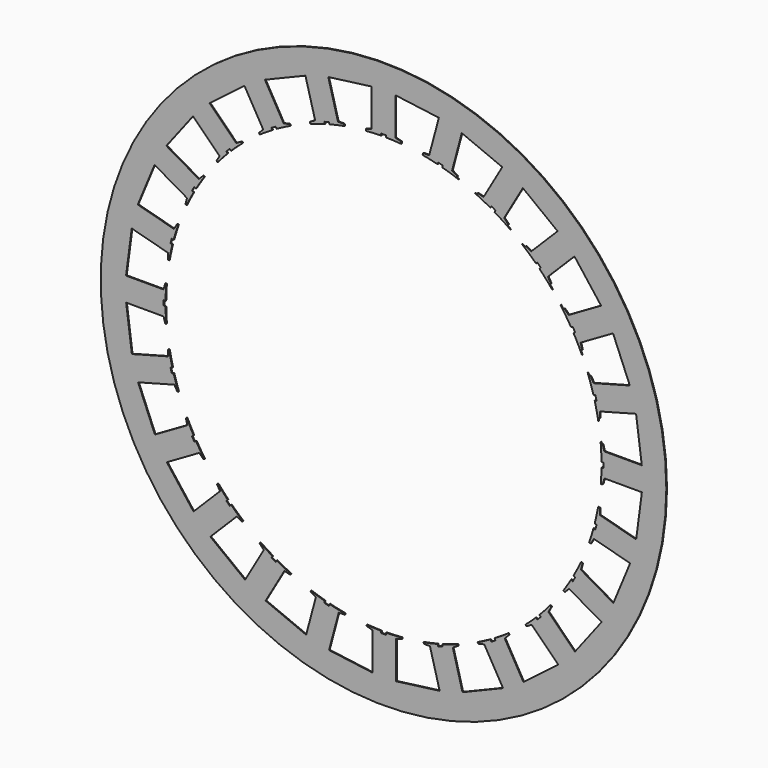
from build123d import *

# Parameters (mm, degrees)
F0_R     = 117.42
F0_R_2   = 90.5
F1_DEPTH = 0.35
F3_DEPTH = 0.351
F5_DEPTH = 0.351


with BuildPart() as f1:
    # F0 (on Front) → F1 (new body)
    with BuildSketch(Plane.XZ):
        Circle(F0_R)
        Circle(F0_R_2, mode=Mode.SUBTRACT)
    extrude(amount=F1_DEPTH)

    # F2 (on face) → F3 (cut, through all)
    with BuildSketch(Plane.XZ.offset(0.35)):
        with BuildLine():
            Line((7.35, 91.001039351), (7.35, 90.201039351))
            ThreePointArc((7.35, 90.201039351), (11.8126203959, 89.7257599543), (16.2461920489, 89.0298334487))
            Line((16.2461920489, 89.0298334487), (16.4532472849, 89.8025741098))
            Line((16.4532472849, 89.8025741098), (18.9519490961, 89.8163312564))
            Line((18.9519490961, 89.8163312564), (22.9791734379, 104.8461371135))
            Line((22.9791734379, 104.8461371135), (13.9595867189, 106.0335882322))
            Line((13.9595867189, 106.0335882322), (4.94, 107.221039351))
            Line((4.94, 107.221039351), (4.94, 91.661039351))
            Line((4.94, 91.661039351), (7.35, 91.001039351))
        make_face()
        with BuildLine():
            ThreePointArc((-16.2168209482, 89.0351880906), (-11.7768900226, 89.7304567101), (-7.3079183955, 90.2044584748))
            Line((-7.3079183955, 90.2044584748), (-7.3079183955, 90.9589577465))
            Line((-7.3079183955, 90.9589577465), (-4.8979183955, 91.6189577465))
            Line((-4.8979183955, 91.6189577465), (-4.8979183955, 107.1789577465))
            Line((-4.8979183955, 107.1789577465), (-13.9175051144, 105.9915066277))
            Line((-13.9175051144, 105.9915066277), (-22.9370918333, 104.804055509))
            Line((-22.9370918333, 104.804055509), (-18.9098674915, 89.7742496519))
            Line((-18.9098674915, 89.7742496519), (-16.4111656804, 89.7604925052))
            Line((-16.4111656804, 89.7604925052), (-16.2168209482, 89.0351880906))
        make_face()
        with BuildLine():
            ThreePointArc((-38.6942784312, 81.8107744535), (-34.5786193429, 83.6335404269), (-30.3774193068, 85.2494128792))
            Line((-30.3774193068, 85.2494128792), (-30.5587360975, 85.9260963543))
            Line((-30.5587360975, 85.9260963543), (-28.4016754259, 87.1873612984))
            Line((-28.4016754259, 87.1873612984), (-32.4288997677, 102.2171671554))
            Line((-32.4288997677, 102.2171671554), (-40.8338165573, 98.7357366305))
            Line((-40.8338165573, 98.7357366305), (-49.2387333469, 95.2543061057))
            Line((-49.2387333469, 95.2543061057), (-41.4587333469, 81.7789508228))
            Line((-41.4587333469, 81.7789508228), (-39.0416121238, 82.4123740563))
            Line((-39.0416121238, 82.4123740563), (-38.6942784312, 81.8107744535))
        make_face()
        with BuildLine():
            ThreePointArc((-58.5499893895, 69.0083237189), (-55.0402014846, 71.8388907246), (-51.3937868632, 74.491131498))
            Line((-51.3937868632, 74.491131498), (-51.7147010186, 75.04697112))
            Line((-51.7147010186, 75.04697112), (-49.9575797955, 76.8235478865))
            Line((-49.9575797955, 76.8235478865), (-57.7375797955, 90.2989031694))
            Line((-57.7375797955, 90.2989031694), (-64.9550454664, 84.7607469753))
            Line((-64.9550454664, 84.7607469753), (-72.1725111372, 79.2225907813))
            Line((-72.1725111372, 79.2225907813), (-61.1699296219, 68.220009266))
            Line((-61.1699296219, 68.220009266), (-58.9991118037, 69.4574461331))
            Line((-58.9991118037, 69.4574461331), (-58.5499893895, 69.0083237189))
        make_face()
        with BuildLine():
            ThreePointArc((-74.4244093249, 51.4903612013), (-71.7627334883, 55.139460301), (-68.9223095649, 58.6512169033))
            Line((-68.9223095649, 58.6512169033), (-69.3340691113, 59.0629764496))
            Line((-69.3340691113, 59.0629764496), (-68.0966322442, 61.2337942679))
            Line((-68.0966322442, 61.2337942679), (-79.0992137595, 72.2363757831))
            Line((-79.0992137595, 72.2363757831), (-84.6373699535, 65.0189101123))
            Line((-84.6373699535, 65.0189101123), (-90.1755261476, 57.8014444414))
            Line((-90.1755261476, 57.8014444414), (-76.7001708647, 50.0214444414))
            Line((-76.7001708647, 50.0214444414), (-74.9235940982, 51.7785656646))
            Line((-74.9235940982, 51.7785656646), (-74.4244093249, 51.4903612013))
        make_face()
        with BuildLine():
            ThreePointArc((-85.2251934857, 30.4453016953), (-83.5973003854, 34.6661415256), (-81.7605171259, 38.8003587523))
            Line((-81.7605171259, 38.8003587523), (-82.2161095574, 39.0633951652))
            Line((-82.2161095574, 39.0633951652), (-81.5826863239, 41.4805163883))
            Line((-81.5826863239, 41.4805163883), (-95.0580416068, 49.2605163883))
            Line((-95.0580416068, 49.2605163883), (-98.5394721316, 40.8555995987))
            Line((-98.5394721316, 40.8555995987), (-102.0209026565, 32.4506828091))
            Line((-102.0209026565, 32.4506828091), (-86.9910967994, 28.4234584673))
            Line((-86.9910967994, 28.4234584673), (-85.7298318554, 30.5805191389))
            Line((-85.7298318554, 30.5805191389), (-85.2251934857, 30.4453016953))
        make_face()
        with BuildLine():
            ThreePointArc((-90.2044584748, 7.3079183955), (-89.7257599543, 11.8126203959), (-89.022244548, 16.2877246918))
            Line((-89.022244548, 16.2877246918), (-89.4829325891, 16.4111656804))
            Line((-89.4829325891, 16.4111656804), (-89.4966897357, 18.9098674915))
            Line((-89.4966897357, 18.9098674915), (-104.5264955928, 22.9370918333))
            Line((-104.5264955928, 22.9370918333), (-105.7139467115, 13.9175051144))
            Line((-105.7139467115, 13.9175051144), (-106.9013978303, 4.8979183955))
            Line((-106.9013978303, 4.8979183955), (-91.3413978303, 4.8979183955))
            Line((-91.3413978303, 4.8979183955), (-90.6813978303, 7.3079183955))
            Line((-90.6813978303, 7.3079183955), (-90.2044584748, 7.3079183955))
        make_face()
        with BuildLine():
            ThreePointArc((-89.0129240771, -16.3385846157), (-89.7196178951, -11.8591806104), (-90.201039351, -7.35))
            Line((-90.201039351, -7.35), (-90.6393162258, -7.35))
            Line((-90.6393162258, -7.35), (-91.2993162258, -4.94))
            Line((-91.2993162258, -4.94), (-106.8593162258, -4.94))
            Line((-106.8593162258, -4.94), (-105.671865107, -13.9595867189))
            Line((-105.671865107, -13.9595867189), (-104.4844139883, -22.9791734379))
            Line((-104.4844139883, -22.9791734379), (-89.4546081312, -18.9519490961))
            Line((-89.4546081312, -18.9519490961), (-89.4408509845, -16.4532472849))
            Line((-89.4408509845, -16.4532472849), (-89.0129240771, -16.3385846157))
        make_face()
        with BuildLine():
            ThreePointArc((-81.7263916861, -38.8721867403), (-83.5721438112, -34.7267444314), (-85.2077832778, -30.4939939806))
            Line((-85.2077832778, -30.4939939806), (-85.6064548336, -30.6008177021))
            Line((-85.6064548336, -30.6008177021), (-86.8677197777, -28.4437570305))
            Line((-86.8677197777, -28.4437570305), (-101.8975256347, -32.4709813723))
            Line((-101.8975256347, -32.4709813723), (-98.4160951098, -40.8758981619))
            Line((-98.4160951098, -40.8758981619), (-94.934664585, -49.2808149515))
            Line((-94.934664585, -49.2808149515), (-81.4593093021, -41.5008149515))
            Line((-81.4593093021, -41.5008149515), (-82.0927325356, -39.0836937284))
            Line((-82.0927325356, -39.0836937284), (-81.7263916861, -38.8721867403))
        make_face()
        with BuildLine():
            ThreePointArc((-68.8420326491, -58.7454214449), (-71.7007538884, -55.2200316175), (-74.3791286312, -51.5557487005))
            Line((-74.3791286312, -51.5557487005), (-74.7273295993, -51.7567826232))
            Line((-74.7273295993, -51.7567826232), (-76.5039063658, -49.9996614))
            Line((-76.5039063658, -49.9996614), (-89.9792616487, -57.7796614))
            Line((-89.9792616487, -57.7796614), (-84.4411054546, -64.9971270709))
            Line((-84.4411054546, -64.9971270709), (-78.9029492606, -72.2145927417))
            Line((-78.9029492606, -72.2145927417), (-67.9003677453, -61.2120112265))
            Line((-67.9003677453, -61.2120112265), (-69.1378046124, -59.0411934082))
            Line((-69.1378046124, -59.0411934082), (-68.8420326491, -58.7454214449))
        make_face()
        with BuildLine():
            ThreePointArc((-51.2443456156, -74.5940147896), (-54.9189774066, -71.9316058532), (-58.4555358366, -69.0883516235))
            Line((-58.4555358366, -69.0883516235), (-58.7433349289, -69.3761507158))
            Line((-58.7433349289, -69.3761507158), (-60.9141527472, -68.1387138487))
            Line((-60.9141527472, -68.1387138487), (-71.9167342624, -79.141295364))
            Line((-71.9167342624, -79.141295364), (-64.6992685916, -84.6794515581))
            Line((-64.6992685916, -84.6794515581), (-57.4818029207, -90.2176077521))
            Line((-57.4818029207, -90.2176077521), (-49.7018029207, -76.7422524692))
            Line((-49.7018029207, -76.7422524692), (-51.4589241439, -74.9656757027))
            Line((-51.4589241439, -74.9656757027), (-51.2443456156, -74.5940147896))
        make_face()
        with BuildLine():
            ThreePointArc((-30.143145351, -85.3325306571), (-34.3798043636, -83.7154648313), (-38.5301421361, -81.8882051762))
            Line((-38.5301421361, -81.8882051762), (-38.7437536445, -82.2581911619))
            Line((-38.7437536445, -82.2581911619), (-41.1608748676, -81.6247679284))
            Line((-41.1608748676, -81.6247679284), (-48.9408748676, -95.1001232113))
            Line((-48.9408748676, -95.1001232113), (-40.535958078, -98.5815537362))
            Line((-40.535958078, -98.5815537362), (-32.1310412884, -102.062984261))
            Line((-32.1310412884, -102.062984261), (-28.1038169466, -87.033178404))
            Line((-28.1038169466, -87.033178404), (-30.2608776182, -85.7719134599))
            Line((-30.2608776182, -85.7719134599), (-30.143145351, -85.3325306571))
        make_face()
        with BuildLine():
            ThreePointArc((-6.9882768748, -90.2297843637), (-11.4946009779, -89.7670549164), (-15.9721247912, -89.079409684))
            Line((-15.9721247912, -89.079409684), (-16.0915241597, -89.5250141936))
            Line((-16.0915241597, -89.5250141936), (-18.5902259708, -89.5387713403))
            Line((-18.5902259708, -89.5387713403), (-22.6174503126, -104.5685771973))
            Line((-22.6174503126, -104.5685771973), (-13.5978635937, -105.7560283161))
            Line((-13.5978635937, -105.7560283161), (-4.5782768748, -106.9434794348))
            Line((-4.5782768748, -106.9434794348), (-4.5782768748, -91.3834794348))
            Line((-4.5782768748, -91.3834794348), (-6.9882768748, -90.7234794348))
            Line((-6.9882768748, -90.7234794348), (-6.9882768748, -90.2297843637))
        make_face()
        with BuildLine():
            Line((16.7728888056, -89.4829325891), (16.6323669842, -88.9584980117))
            ThreePointArc((16.6323669842, -88.9584980117), (12.1662041269, -89.6785006406), (7.6696415207, -90.1744231972))
            Line((7.6696415207, -90.1744231972), (7.6696415207, -90.6813978303))
            Line((7.6696415207, -90.6813978303), (5.2596415207, -91.3413978303))
            Line((5.2596415207, -91.3413978303), (5.2596415207, -106.9013978303))
            Line((5.2596415207, -106.9013978303), (14.2792282396, -105.7139467115))
            Line((14.2792282396, -105.7139467115), (23.2988149586, -104.5264955928))
            Line((23.2988149586, -104.5264955928), (19.2715906168, -89.4966897357))
            Line((19.2715906168, -89.4966897357), (16.7728888056, -89.4829325891))
        make_face()
        with BuildLine():
            Line((39.4033352491, -82.1348141401), (39.1037189264, -81.6158634465))
            ThreePointArc((39.1037189264, -81.6158634465), (34.9830509393, -83.4651792484), (30.7752488822, -85.1066040695))
            Line((30.7752488822, -85.1066040695), (30.9204592228, -85.6485364381))
            Line((30.9204592228, -85.6485364381), (28.7633985512, -86.9098013822))
            Line((28.7633985512, -86.9098013822), (32.790622893, -101.9396072392))
            Line((32.790622893, -101.9396072392), (41.1955396826, -98.4581767144))
            Line((41.1955396826, -98.4581767144), (49.6004564722, -94.9767461895))
            Line((49.6004564722, -94.9767461895), (41.8204564722, -81.5013909066))
            Line((41.8204564722, -81.5013909066), (39.4033352491, -82.1348141401))
        make_face()
        with BuildLine():
            Line((59.3608349289, -69.1798862169), (58.8950318574, -68.7140831454))
            ThreePointArc((58.8950318574, -68.7140831454), (55.3995226584, -71.5621610156), (51.7664987786, -74.2326047246))
            Line((51.7664987786, -74.2326047246), (52.0764241439, -74.7694112038))
            Line((52.0764241439, -74.7694112038), (50.3193029207, -76.5459879703))
            Line((50.3193029207, -76.5459879703), (58.0993029207, -90.0213432532))
            Line((58.0993029207, -90.0213432532), (65.3167685916, -84.4831870592))
            Line((65.3167685916, -84.4831870592), (72.5342342624, -78.9450308651))
            Line((72.5342342624, -78.9450308651), (61.5316527472, -67.9424493498))
            Line((61.5316527472, -67.9424493498), (59.3608349289, -69.1798862169))
        make_face()
        with BuildLine():
            Line((75.2853172234, -51.5010057484), (74.66401667, -51.1422977066))
            ThreePointArc((74.6640166699, -51.1422977066), (72.0288036264, -54.7914359015), (69.2154099771, -58.3050342741))
            Line((69.2154099771, -58.3050342741), (69.6957922365, -58.7854165335))
            Line((69.6957922365, -58.7854165335), (68.4583553694, -60.9562343517))
            Line((68.4583553694, -60.9562343517), (79.4609368847, -71.958815867))
            Line((79.4609368847, -71.958815867), (84.9990930788, -64.7413501961))
            Line((84.9990930788, -64.7413501961), (90.5372492728, -57.5238845253))
            Line((90.5372492728, -57.5238845253), (77.0618939899, -49.7438845253))
            Line((77.0618939899, -49.7438845253), (75.2853172234, -51.5010057484))
        make_face()
        with BuildLine():
            Line((86.0915549806, -30.3029592228), (85.3465798698, -30.1033437434))
            ThreePointArc((85.3465798698, -30.1033437434), (83.7469654157, -34.3029996306), (81.9408440386, -38.418069684))
            Line((81.9408440386, -38.418069684), (82.5778326826, -38.7858352491))
            Line((82.5778326826, -38.7858352491), (81.9444094491, -41.2029564722))
            Line((81.9444094491, -41.2029564722), (95.419764732, -48.9829564722))
            Line((95.419764732, -48.9829564722), (98.9011952569, -40.5780396826))
            Line((98.9011952569, -40.5780396826), (102.3826257817, -32.173122893))
            Line((102.3826257817, -32.173122893), (87.3528199247, -28.1458985512))
            Line((87.3528199247, -28.1458985512), (86.0915549806, -30.3029592228))
        make_face()
        with BuildLine():
            Line((90.2431209555, -7.0303584793), (90.201039351, -7.35))
            ThreePointArc((90.201039351, -7.35), (89.7465520631, -11.6535999923), (89.0868535315, -15.9305532813))
            Line((89.0868535315, -15.9305532813), (89.8446557143, -16.1336057642))
            Line((89.8446557143, -16.1336057642), (89.858412861, -18.6323075754))
            Line((89.858412861, -18.6323075754), (104.888218718, -22.6595319172))
            Line((104.888218718, -22.6595319172), (106.0756698368, -13.6399451982))
            Line((106.0756698368, -13.6399451982), (107.2631209555, -4.6203584793))
            Line((107.2631209555, -4.6203584793), (91.7031209555, -4.6203584793))
            Line((91.7031209555, -4.6203584793), (91.0431209555, -7.0303584793))
            Line((91.0431209555, -7.0303584793), (90.2431209555, -7.0303584793))
        make_face()
        with BuildLine():
            Line((89.0298334487, 16.523751965), (89.1703911715, 15.4561100644))
            ThreePointArc((89.1703911715, 15.4561100644), (89.7257599543, 11.8126203959), (90.1323194207, 8.1495396093))
            Line((90.1323194207, 8.1495396093), (90.201039351, 7.6275599162))
            Line((90.201039351, 7.6275599162), (91.001039351, 7.6275599162))
            Line((91.001039351, 7.6275599162), (91.661039351, 5.2175599162))
            Line((91.661039351, 5.2175599162), (107.221039351, 5.2175599162))
            Line((107.221039351, 5.2175599162), (106.0335882322, 14.2371466351))
            Line((106.0335882322, 14.2371466351), (104.8461371135, 23.256733354))
            Line((104.8461371135, 23.256733354), (89.8163312564, 19.2295090122))
            Line((89.8163312564, 19.2295090122), (89.8025741098, 16.7308072011))
            Line((89.8025741098, 16.7308072011), (89.0298334487, 16.523751965))
        make_face()
        with BuildLine():
            Line((81.7616353378, 38.9612536445), (82.38587068, 37.4542162152))
            ThreePointArc((82.38587068, 37.4542162152), (83.6110976923, 34.632850629), (84.7397381016, 31.771477562))
            Line((84.7397381016, 31.771477562), (85.1954372978, 30.6713223821))
            Line((85.1954372978, 30.6713223821), (85.9681779588, 30.8783776182))
            Line((85.9681779588, 30.8783776182), (87.2294429029, 28.7213169466))
            Line((87.2294429029, 28.7213169466), (102.2592487599, 32.7485412884))
            Line((102.2592487599, 32.7485412884), (98.7778182351, 41.153458078))
            Line((98.7778182351, 41.153458078), (95.2963877102, 49.5583748676))
            Line((95.2963877102, 49.5583748676), (81.8210324273, 41.7783748676))
            Line((81.8210324273, 41.7783748676), (82.4544556608, 39.3612536445))
            Line((82.4544556608, 39.3612536445), (81.7616353378, 38.9612536445))
        make_face()
        with BuildLine():
            Line((68.9338423127, 58.7530678995), (70.0356048307, 57.3172230311))
            ThreePointArc((70.0356048307, 57.3172230311), (71.7984772964, 55.0929093253), (73.4907343824, 52.8144105329))
            Line((73.4907343824, 52.8144105329), (74.3962324015, 51.6343425393))
            Line((74.3962324015, 51.6343425393), (75.0890527245, 52.0343425393))
            Line((75.0890527245, 52.0343425393), (76.865629491, 50.2772213162))
            Line((76.865629491, 50.2772213162), (90.3409847739, 58.0572213162))
            Line((90.3409847739, 58.0572213162), (84.8028285799, 65.2746869871))
            Line((84.8028285799, 65.2746869871), (79.2646723858, 72.4921526579))
            Line((79.2646723858, 72.4921526579), (68.2620908705, 61.4895711426))
            Line((68.2620908705, 61.4895711426), (69.4995277376, 59.3187533244))
            Line((69.4995277376, 59.3187533244), (68.9338423127, 58.7530678995))
        make_face()
        with BuildLine():
            Line((51.4206472691, 74.5504152959), (52.6211488142, 73.6292380612))
            ThreePointArc((52.6211488142, 73.6292380612), (55.0929093253, 71.7984772964), (57.501027125, 69.8847757353))
            Line((57.501027125, 69.8847757353), (58.5393726292, 69.088025207))
            Line((58.5393726292, 69.088025207), (59.1050580542, 69.653710632))
            Line((59.1050580542, 69.653710632), (61.2758758724, 68.4162737649))
            Line((61.2758758724, 68.4162737649), (72.2784573877, 79.4188552802))
            Line((72.2784573877, 79.4188552802), (65.0609917168, 84.9570114742))
            Line((65.0609917168, 84.9570114742), (57.843526046, 90.4951676683))
            Line((57.843526046, 90.4951676683), (50.063526046, 77.0198123854))
            Line((50.063526046, 77.0198123854), (51.8206472691, 75.2432356189))
            Line((51.8206472691, 75.2432356189), (51.4206472691, 74.5504152959))
        make_face()
        with BuildLine():
            Line((30.4155455074, 85.2767327151), (31.1998116263, 84.9518790521))
            ThreePointArc((31.1998116263, 84.9518790521), (34.632850629, 83.6110976923), (38.0084513796, 82.131648125))
            Line((38.0084513796, 82.131648125), (38.7054767698, 81.8429307551))
            Line((38.7054767698, 81.8429307551), (39.1054767698, 82.5357510781))
            Line((39.1054767698, 82.5357510781), (41.5225979929, 81.9023278446))
            Line((41.5225979929, 81.9023278446), (49.3025979929, 95.3776831275))
            Line((49.3025979929, 95.3776831275), (40.8976812033, 98.8591136523))
            Line((40.8976812033, 98.8591136523), (32.4927644137, 102.3405441772))
            Line((32.4927644137, 102.3405441772), (28.4655400719, 87.3107383202))
            Line((28.4655400719, 87.3107383202), (30.6226007435, 86.0494733761))
            Line((30.6226007435, 86.0494733761), (30.4155455074, 85.2767327151))
        make_face()
    extrude(amount=-F3_DEPTH, mode=Mode.SUBTRACT)

    # F4 (on face) → F5 (cut, through all)
    with BuildSketch(Plane.XZ.offset(0.35)):
        with BuildLine():
            ThreePointArc((-1, 90.4944749695), (0, 90.5), (1, 90.4944749695))
            Line((1, 90.4944749695), (1, 91.3))
            Line((1, 91.3), (-1, 91.3))
            Line((-1, 91.3), (-1, 90.4944749695))
        make_face()
        with BuildLine():
            Line((22.6642529916, 88.4478469853), (22.4557677724, 87.6697695546))
            ThreePointArc((22.4557677724, 87.6697695546), (23.4231235818, 87.4162872792), (24.3876194249, 87.1521314644))
            Line((24.3876194249, 87.1521314644), (24.5961046441, 87.9302088951))
            Line((24.5961046441, 87.9302088951), (22.6642529916, 88.4478469853))
        make_face()
        with BuildLine():
            ThreePointArc((-24.3876194249, 87.1521314644), (-23.4231235818, 87.4162872792), (-22.4557677724, 87.6697695546))
            Line((-22.4557677724, 87.6697695546), (-22.6642529916, 88.4478469853))
            Line((-22.6642529916, 88.4478469853), (-24.5961046441, 87.9302088951))
            Line((-24.5961046441, 87.9302088951), (-24.3876194249, 87.1521314644))
        make_face()
        with BuildLine():
            ThreePointArc((-46.1132628885, 77.8705142257), (-45.25, 78.3752990425), (-44.381212081, 78.8705142257))
            Line((-44.381212081, 78.8705142257), (-44.7839745962, 79.5681193655))
            Line((-44.7839745962, 79.5681193655), (-46.5160254038, 78.5681193655))
            Line((-46.5160254038, 78.5681193655), (-46.1132628885, 77.8705142257))
        make_face()
        with BuildLine():
            Line((44.7839745962, 79.5681193655), (44.381212081, 78.8705142257))
            ThreePointArc((44.381212081, 78.8705142257), (45.25, 78.3752990425), (46.1132628885, 77.8705142257))
            Line((46.1132628885, 77.8705142257), (46.5160254038, 78.5681193655))
            Line((46.5160254038, 78.5681193655), (44.7839745962, 79.5681193655))
        make_face()
        with BuildLine():
            ThreePointArc((-64.696363692, 63.2821501296), (-63.9931636974, 63.9931636974), (-63.2821501296, 64.696363692))
            Line((-63.2821501296, 64.696363692), (-63.8517423411, 65.2659559035))
            Line((-63.8517423411, 65.2659559035), (-65.2659559035, 63.8517423411))
            Line((-65.2659559035, 63.8517423411), (-64.696363692, 63.2821501296))
        make_face()
        with BuildLine():
            Line((63.8517423411, 65.2659559035), (63.2821501296, 64.696363692))
            ThreePointArc((63.2821501296, 64.696363692), (63.9931636974, 63.9931636974), (64.696363692, 63.2821501296))
            Line((64.696363692, 63.2821501296), (65.2659559035, 63.8517423411))
            Line((65.2659559035, 63.8517423411), (63.8517423411, 65.2659559035))
        make_face()
        with BuildLine():
            ThreePointArc((-78.8705142257, 44.381212081), (-78.3752990425, 45.25), (-77.8705142257, 46.1132628885))
            Line((-77.8705142257, 46.1132628885), (-78.5681193655, 46.5160254038))
            Line((-78.5681193655, 46.5160254038), (-79.5681193655, 44.7839745962))
            Line((-79.5681193655, 44.7839745962), (-78.8705142257, 44.381212081))
        make_face()
        with BuildLine():
            Line((78.5681193655, 46.5160254038), (77.8705142257, 46.1132628885))
            ThreePointArc((77.8705142257, 46.1132628885), (78.3752990425, 45.25), (78.8705142257, 44.381212081))
            Line((78.8705142257, 44.381212081), (79.5681193655, 44.7839745962))
            Line((79.5681193655, 44.7839745962), (78.5681193655, 46.5160254038))
        make_face()
        with BuildLine():
            ThreePointArc((-87.6697695546, 22.4557677724), (-87.4162872792, 23.4231235818), (-87.1521314644, 24.3876194249))
            Line((-87.1521314644, 24.3876194249), (-87.9302088951, 24.5961046441))
            Line((-87.9302088951, 24.5961046441), (-88.4478469853, 22.6642529916))
            Line((-88.4478469853, 22.6642529916), (-87.6697695546, 22.4557677724))
        make_face()
        with BuildLine():
            Line((87.9302088951, 24.5961046441), (87.1521314644, 24.3876194249))
            ThreePointArc((87.1521314644, 24.3876194249), (87.4162872792, 23.4231235818), (87.6697695546, 22.4557677724))
            Line((87.6697695546, 22.4557677724), (88.4478469853, 22.6642529916))
            Line((88.4478469853, 22.6642529916), (87.9302088951, 24.5961046441))
        make_face()
        with BuildLine():
            ThreePointArc((-90.4944749695, -1), (-90.5, 0), (-90.4944749695, 1))
            Line((-90.4944749695, 1), (-91.3, 1))
            Line((-91.3, 1), (-91.3, -1))
            Line((-91.3, -1), (-90.4944749695, -1))
        make_face()
        with BuildLine():
            Line((91.3, 1), (90.4944749695, 1))
            ThreePointArc((90.4944749695, 1), (90.5, 0), (90.4944749695, -1))
            Line((90.4944749695, -1), (91.3, -1))
            Line((91.3, -1), (91.3, 1))
        make_face()
        with BuildLine():
            ThreePointArc((-87.1521314644, -24.3876194249), (-87.4162872792, -23.4231235818), (-87.6697695546, -22.4557677724))
            Line((-87.6697695546, -22.4557677724), (-88.4478469853, -22.6642529916))
            Line((-88.4478469853, -22.6642529916), (-87.9302088951, -24.5961046441))
            Line((-87.9302088951, -24.5961046441), (-87.1521314644, -24.3876194249))
        make_face()
        with BuildLine():
            ThreePointArc((-77.8705142257, -46.1132628885), (-78.3752990425, -45.25), (-78.8705142257, -44.381212081))
            Line((-78.8705142257, -44.381212081), (-79.5681193655, -44.7839745962))
            Line((-79.5681193655, -44.7839745962), (-78.5681193655, -46.5160254038))
            Line((-78.5681193655, -46.5160254038), (-77.8705142257, -46.1132628885))
        make_face()
        with BuildLine():
            Line((88.4478469853, -22.6642529916), (87.6697695546, -22.4557677724))
            ThreePointArc((87.6697695546, -22.4557677724), (87.4162872792, -23.4231235818), (87.1521314644, -24.3876194249))
            Line((87.1521314644, -24.3876194249), (87.9302088951, -24.5961046441))
            Line((87.9302088951, -24.5961046441), (88.4478469853, -22.6642529916))
        make_face()
        with BuildLine():
            ThreePointArc((-63.2821501296, -64.696363692), (-63.9931636974, -63.9931636974), (-64.696363692, -63.2821501296))
            Line((-64.696363692, -63.2821501296), (-65.2659559035, -63.8517423411))
            Line((-65.2659559035, -63.8517423411), (-63.8517423411, -65.2659559035))
            Line((-63.8517423411, -65.2659559035), (-63.2821501296, -64.696363692))
        make_face()
        with BuildLine():
            Line((79.5681193655, -44.7839745962), (78.8705142257, -44.381212081))
            ThreePointArc((78.8705142257, -44.381212081), (78.3752990425, -45.25), (77.8705142257, -46.1132628885))
            Line((77.8705142257, -46.1132628885), (78.5681193655, -46.5160254038))
            Line((78.5681193655, -46.5160254038), (79.5681193655, -44.7839745962))
        make_face()
        with BuildLine():
            ThreePointArc((-44.381212081, -78.8705142257), (-45.25, -78.3752990425), (-46.1132628885, -77.8705142257))
            Line((-46.1132628885, -77.8705142257), (-46.5160254038, -78.5681193655))
            Line((-46.5160254038, -78.5681193655), (-44.7839745962, -79.5681193655))
            Line((-44.7839745962, -79.5681193655), (-44.381212081, -78.8705142257))
        make_face()
        with BuildLine():
            Line((65.2659559035, -63.8517423411), (64.696363692, -63.2821501296))
            ThreePointArc((64.696363692, -63.2821501296), (63.9931636974, -63.9931636974), (63.2821501296, -64.696363692))
            Line((63.2821501296, -64.696363692), (63.8517423411, -65.2659559035))
            Line((63.8517423411, -65.2659559035), (65.2659559035, -63.8517423411))
        make_face()
        with BuildLine():
            ThreePointArc((-22.4557677724, -87.6697695546), (-23.4231235818, -87.4162872792), (-24.3876194249, -87.1521314644))
            Line((-24.3876194249, -87.1521314644), (-24.5961046441, -87.9302088951))
            Line((-24.5961046441, -87.9302088951), (-22.6642529916, -88.4478469853))
            Line((-22.6642529916, -88.4478469853), (-22.4557677724, -87.6697695546))
        make_face()
        with BuildLine():
            Line((46.5160254038, -78.5681193655), (46.1132628885, -77.8705142257))
            ThreePointArc((46.1132628885, -77.8705142257), (45.25, -78.3752990425), (44.381212081, -78.8705142257))
            Line((44.381212081, -78.8705142257), (44.7839745962, -79.5681193655))
            Line((44.7839745962, -79.5681193655), (46.5160254038, -78.5681193655))
        make_face()
        with BuildLine():
            ThreePointArc((1, -90.4944749695), (0, -90.5), (-1, -90.4944749695))
            Line((-1, -90.4944749695), (-1, -91.3))
            Line((-1, -91.3), (1, -91.3))
            Line((1, -91.3), (1, -90.4944749695))
        make_face()
        with BuildLine():
            Line((24.5961046441, -87.9302088951), (24.3876194249, -87.1521314644))
            ThreePointArc((24.3876194249, -87.1521314644), (23.4231235818, -87.4162872792), (22.4557677724, -87.6697695546))
            Line((22.4557677724, -87.6697695546), (22.6642529916, -88.4478469853))
            Line((22.6642529916, -88.4478469853), (24.5961046441, -87.9302088951))
        make_face()
    extrude(amount=-F5_DEPTH, mode=Mode.SUBTRACT)


solid = f1.part
